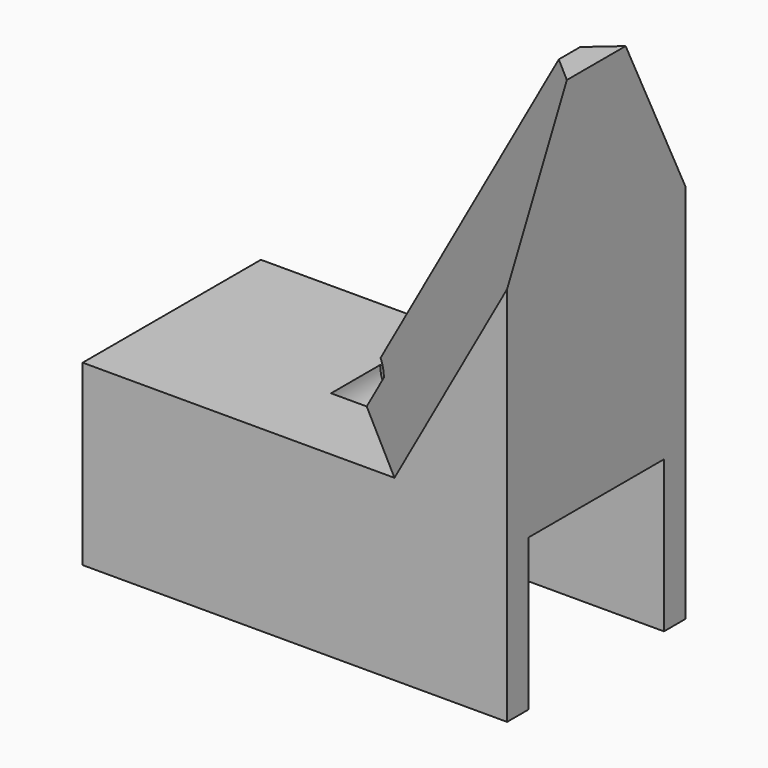
from build123d import *

# Parameters (mm, degrees)
F0_W        = 23.8125
F0_H        = 12.5
F1_DEPTH    = 10
F2_W        = 9.5
F2_H        = 8.5
F3_DEPTH    = 23.8135
F4_W        = 11.5
F4_H        = 12.5
F5_DEPTH    = 20
F6_SIZE2    = 18
F6_SIZE     = 10
F7_T4_DEPTH = 48.8797731496
F7_T9_DEPTH = 48.8797731496
F8_W        = 2
F8_H        = 3.4425717247


# Not quite as in the source:
# - a fillet or chamfer that OpenCascade refuses, or shapes differently, is made with other operations: its cross-section is extruded or revolved along the edge and cut away or added


with BuildPart() as f1:
    # F0 (on Top) → F1 (new body)
    with BuildSketch(Plane.XY):
        with Locations((-12.5924281826, 6.2716105528)):
            Rectangle(F0_W, F0_H)
    extrude(amount=F1_DEPTH)

    # F2 (on face) → F3 (cut, through all)
    with BuildSketch(Plane.YZ.offset(-0.6861781826)):
        with Locations((6.2716105528, 4.25)):
            Rectangle(F2_W, F2_H)
    extrude(amount=-F3_DEPTH, mode=Mode.SUBTRACT)

    # F4 (on face) → F5 (join)
    with BuildSketch(Plane.XY.offset(10)):
        with Locations((-6.4361781826, 6.2716105528)):
            Rectangle(F4_W, F4_H)
    extrude(amount=F5_DEPTH)

    # F6
    f6_edges = [f1.edges().sort_by_distance(p)[0] for p in [
        (-12.186178, 6.271611, 30),
    ]]
    f6_side = f1.faces().sort_by_distance((-6.436178, 6.271611, 30))[0]
    chamfer(f6_edges, length=F6_SIZE, length2=F6_SIZE2, reference=f6_side)

    # F7: chamfer of 5.5 on 2 edges, made by hand


with BuildPart() as f7_tool2:
    # F7_s3 → F7_t4 (new body)
    with BuildSketch(Plane(origin=(19.0892991485, 0, 34.3607384673), x_dir=(0, 1, 0), z_dir=(-0.4856429312, 0, -0.8741572761))):
        Polygon((12.5216105528, -10.9803515006), (7.0216105528, -16.4803515006), (12.5216105528, -16.4803515006), align=None)
    extrude(amount=F7_T4_DEPTH)

    split(bisect_by=Plane.XY.offset(10), keep=Keep.TOP)


with BuildPart() as f1_1:
    add(f1.part)

    # F7_t1: cut F7_tool2
    add(f7_tool2.part, mode=Mode.SUBTRACT)


with BuildPart() as f7_tool7:
    # F7_s8 → F7_t9 (new body)
    with BuildSketch(Plane(origin=(19.0892991485, 0, 34.3607384673), x_dir=(0, 1, 0), z_dir=(-0.4856429312, 0, -0.8741572761))):
        Polygon((5.5216105528, -16.4803515006), (0.0216105528, -10.9803515006), (0.0216105528, -16.4803515006), align=None)
    extrude(amount=F7_T9_DEPTH)

    split(bisect_by=Plane.XY.offset(10), keep=Keep.TOP)


with BuildPart() as f1_2:
    add(f1_1.part)

    # F7_t6: cut F7_tool7
    add(f7_tool7.part, mode=Mode.SUBTRACT)

    # F8 (on face) → F9 (revolve, cut)
    with BuildSketch(Plane.XY.offset(10)):
        with Locations((-11.1861781826, 6.2716105528)):
            Rectangle(F8_W, F8_H)
    revolve(axis=Axis((-12.1861781826, 6.2716105528, 10), (0, -1, 0)), mode=Mode.SUBTRACT)


solid = f1_2.part
